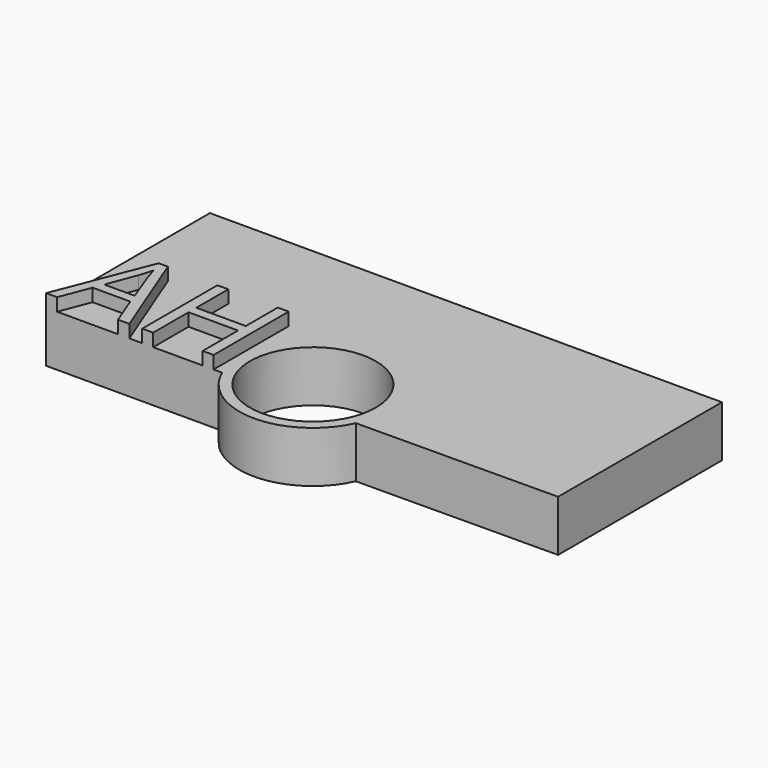
from build123d import *

# Parameters (mm, degrees)
F0_R         = 7.804993174
F1_DEPTH     = 6.35
F2_TEXT_SIZE = 16.3170356374
F3_DEPTH     = 1.5875


# Not quite as in the source:
# - Text() gives the source's letters only with a copy of the font that has no kerning and outlines rounded to 1/6400 em; it was checked with that copy


with BuildPart() as f1:
    # F0 (on Top) → F1 (new body)
    with BuildSketch(Plane.XY):
        with BuildLine():
            Line((13.9085481167, 38.8988703489), (-49.5914518833, 38.8988703489))
            Line((-49.5914518833, 38.8988703489), (-49.5914518833, 13.4988703489))
            Line((-49.5914518833, 13.4988703489), (-27.7623176447, 13.4988703489))
            ThreePointArc((-27.7623176447, 13.4988703489), (-21.1781816678, 26.0154683333), (-10.225958454, 17.0675703489))
            ThreePointArc((-10.225958454, 17.0675703489), (-10.4294698065, 15.1504815256), (-11.0309324569, 13.3188458884))
            Line((-11.0309324569, 13.3188458884), (13.9085481167, 13.4988703489))
            Line((13.9085481167, 13.4988703489), (13.9085481167, 38.8988703489))
        make_face()
        with BuildLine():
            ThreePointArc((-10.225958454, 17.0675703489), (-21.1781816678, 26.0154683333), (-27.7623176447, 13.4988703489))
            ThreePointArc((-27.7623176447, 13.4988703489), (-19.4555026932, 7.9367988722), (-11.0309324569, 13.3188458884))
            ThreePointArc((-11.0309324569, 13.3188458884), (-10.4294698065, 15.1504815256), (-10.225958454, 17.0675703489))
        make_face()
        with Locations((-19.357258454, 17.0675703489)):
            Circle(F0_R, mode=Mode.SUBTRACT)
    extrude(amount=F1_DEPTH)

    # F2 (on face) → F3 (join)
    with BuildSketch(Plane.XY.offset(6.35)):
        with Locations((-49.5914518833, 13.4988703489)):
            Text('AH', F2_TEXT_SIZE, font='Open Sans', text_align=(TextAlign.LEFT, TextAlign.BOTTOM))
    extrude(amount=F3_DEPTH)


solid = f1.part
